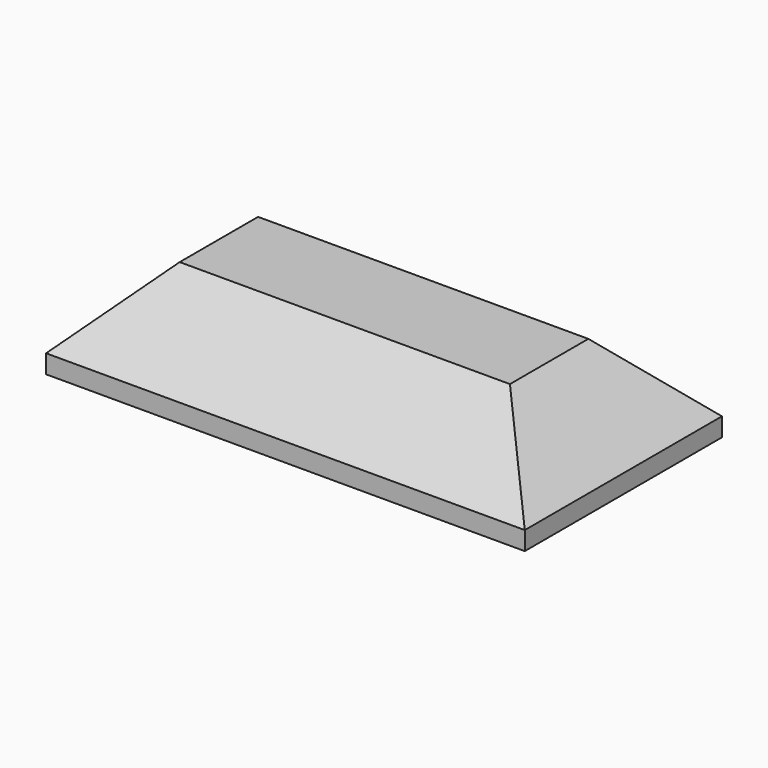
from build123d import *

# Parameters (mm, degrees)
F0_W        = 129.0121003985
F0_H        = 66.4112940431
F1_DEPTH    = 25
F2_R        = 5.1578241127
F3_DEPTH    = 25
F4_T1_DEPTH = 231.8794199172
F4_T3_DEPTH = 169.2786135617


# Not quite as in the source:
# - a fillet or chamfer that OpenCascade refuses, or shapes differently, is made with other operations: its cross-section is extruded or revolved along the edge and cut away or added


with BuildPart() as f1:
    # F0 (on Top) → F1 (new body)
    with BuildSketch(Plane.XY):
        with Locations((1.633066684, 0.4536285996)):
            Rectangle(F0_W, F0_H)
    extrude(amount=F1_DEPTH)

    # F2 (on face) → F3 (cut)
    with BuildSketch(Plane.XY.offset(25)):
        with Locations((-53.4375011921, 2.8125003446)):
            Circle(F2_R)
    extrude(amount=-F3_DEPTH, mode=Mode.SUBTRACT)

    # F4: chamfer of 20 on 4 edges, made by hand

    # F4_s2 → F4_t1 (cut)
    with BuildSketch(Plane.YZ.offset(-114.3066432746)):
        Polygon((-12.7520184219, 25), (-32.7520184219, 5), (-32.7520184219, 25), align=None)
        Polygon((33.6592756212, 5), (13.6592756212, 25), (33.6592756212, 25), align=None)
    extrude(amount=F4_T1_DEPTH, mode=Mode.SUBTRACT)

    # F4_s4 → F4_t3 (cut)
    with BuildSketch(Plane.XZ.offset(-85.0929353805)):
        Polygon((-62.8729835153, 5), (-42.8729835153, 25), (-62.8729835153, 25), align=None)
        Polygon((66.1391168833, 5), (46.1391168833, 25), (66.1391168833, 25), align=None)
    extrude(amount=F4_T3_DEPTH, mode=Mode.SUBTRACT)


solid = f1.part
